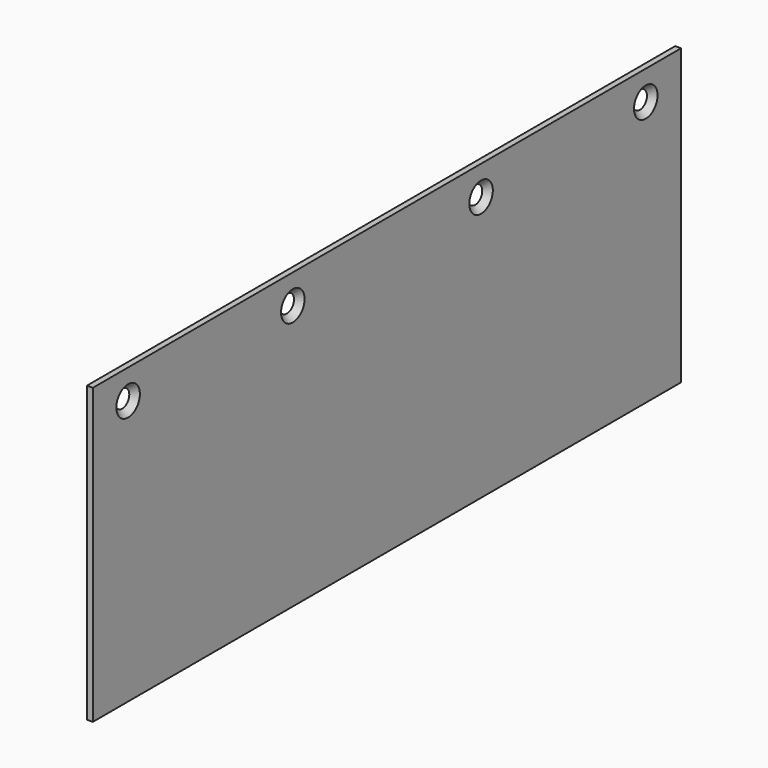
from build123d import *

# Parameters (mm, degrees)
F0_W     = 250
F0_H     = 100
F0_R     = 3
F1_DEPTH = 2
F2_SIZE  = 1.99999


# Not quite as in the source:
# - a fillet or chamfer is up to 0.001 mm smaller than in the source, because OpenCascade refuses the exact size


with BuildPart() as f1:
    # F0 (on Right) → F1 (new body)
    with BuildSketch(Plane.YZ):
        Rectangle(F0_W, F0_H)
        with Locations((-110, 40)):
            Circle(F0_R, mode=Mode.SUBTRACT)
        with Locations((-40, 40)):
            Circle(F0_R, mode=Mode.SUBTRACT)
        with Locations((40, 40)):
            Circle(F0_R, mode=Mode.SUBTRACT)
        with Locations((110, 40)):
            Circle(F0_R, mode=Mode.SUBTRACT)
    extrude(amount=F1_DEPTH)

    # F2 (size 2 in the source; OpenCascade refuses exactly that, so slightly less here)
    f2_edges = [f1.edges().sort_by_distance(p)[0] for p in [
        (2, -113, 40),
        (2, -43, 40),
        (2, 37, 40),
        (2, 107, 40),
    ]]
    chamfer(f2_edges, length=F2_SIZE)


solid = f1.part
